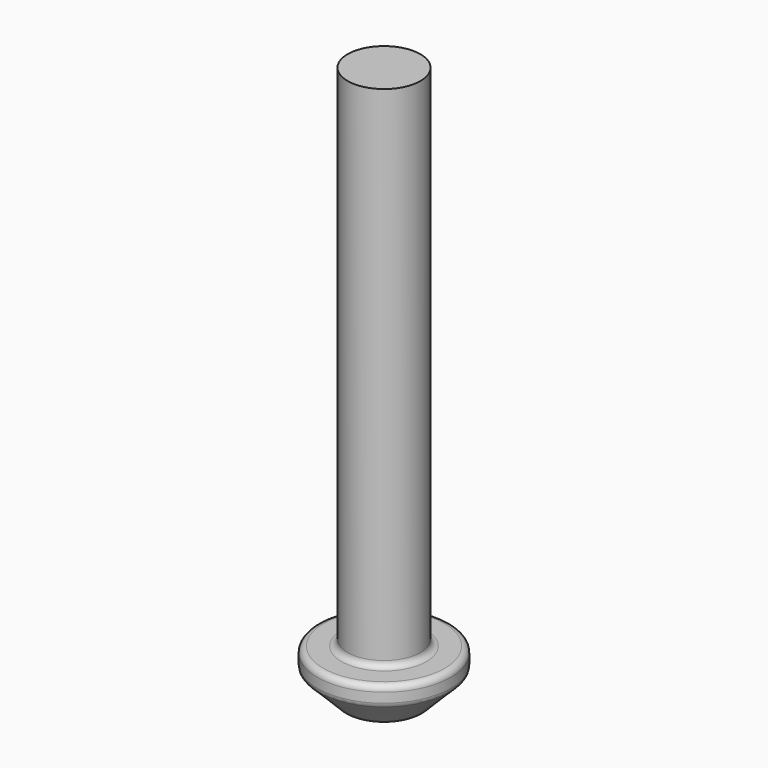
from build123d import *

# Parameters (mm, degrees)
F1_R     = 2.75
F1_R_2   = 1.5
F2_DEPTH = 2
F3_START = 1.5
F3_DEPTH = 0.5
F4_START = 2
F4_DEPTH = 21
F5_SIZE2 = 1.25
F5_SIZE  = 1.25
F6_R     = 0.25


# Not quite as in the source:
# - a feature names something its author has since deleted; it is built from what else it names


with BuildPart() as f2:
    # F1 (on Top) → F2 (new body)
    with BuildSketch(Plane.XY):
        Circle(F1_R)
        Circle(F1_R_2, mode=Mode.SUBTRACT)
        Circle(F1_R_2)
        Polygon((-0.5773502692, -1), (-1.1547005384, 0), (-0.5773502692, 1), (0.5773502692, 1), (1.1547005384, 0), (0.5773502692, -1), align=None, mode=Mode.SUBTRACT)
    extrude(amount=F2_DEPTH)

    # F1 (on Top) → F3 (join)
    with BuildSketch(Plane.XY.offset(F3_START)):
        Polygon((-0.5773502692, 1), (-1.1547005384, 0), (-0.5773502692, -1), (0.5773502692, -1), (1.1547005384, 0), (0.5773502692, 1), align=None)
    extrude(amount=F3_DEPTH)

    # F1 (on Top) → F4 (join)
    with BuildSketch(Plane.XY.offset(F4_START)):
        Circle(F1_R_2)
        Polygon((-0.5773502692, -1), (-1.1547005384, 0), (-0.5773502692, 1), (0.5773502692, 1), (1.1547005384, 0), (0.5773502692, -1), align=None, mode=Mode.SUBTRACT)
        Polygon((-0.5773502692, 1), (-1.1547005384, 0), (-0.5773502692, -1), (0.5773502692, -1), (1.1547005384, 0), (0.5773502692, 1), align=None)
    extrude(amount=F4_DEPTH)

    # F5
    f5_edges = [f2.edges().sort_by_distance(p)[0] for p in [
        (-2.75, 0, 0),
    ]]
    chamfer(f5_edges, length=F5_SIZE, length2=F5_SIZE2)

    # F6
    f6_edges = [f2.edges().sort_by_distance(p)[0] for p in [
        (-2.75, 0, 2),
        (-1.5, 0, 2),
        (-1.5, 0, 0),
        (-2.75, 0, 1.25),
    ]]
    fillet(f6_edges, radius=F6_R)


solid = f2.part
